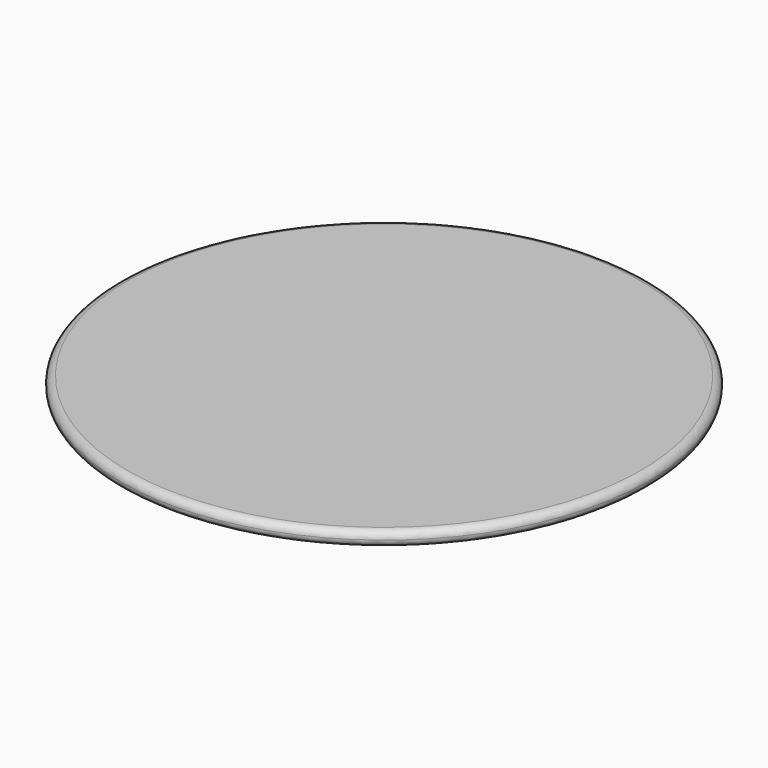
from build123d import *

# Parameters (mm, degrees)
F1_DEPTH = 31.75
F3_DEPTH = 19.05
F4_R     = 19.04999
F5_R     = 6.34999
F6_R     = 8.73125
F7_R     = 8.73125
F8_R     = 8.73125
F9_DEPTH = 19.05


# Not quite as in the source:
# - a fillet or chamfer is up to 0.001 mm smaller than in the source, because OpenCascade refuses the exact size


with BuildPart() as f1:
    # F0 (on Top) → F1 (new body)
    with BuildSketch(Plane.XY):
        with BuildLine():
            add(Edge.make_bspline(
                [(0, -228.6), (395.9468146102, -228.6), (197.9734073051, 114.3), (0, 457.2), (-197.9734073051, 114.3), (-395.9468146102, -228.6), (0, -228.6)],
                knots=[0, 0, 0, 2.0943951024, 2.0943951024, 4.1887902048, 4.1887902048, 6.2831853072, 6.2831853072, 6.2831853072], degree=2, weights=[1, 0.5, 1, 0.5, 1, 0.5, 1]))
        make_face()
    extrude(amount=F1_DEPTH)

    # F2 (on face) → F3 (cut)
    with BuildSketch(Plane(origin=(0, 0, 0), x_dir=(1, 0, 0), z_dir=(0, 0, -1))):
        with BuildLine():
            add(Edge.make_bspline(
                [(0, 228.6), (395.9468146102, 228.6), (197.9734073051, -114.3), (0, -457.2), (-197.9734073051, -114.3), (-395.9468146102, 228.6), (0, 228.6)],
                knots=[0, 0, 0, 2.0943951024, 2.0943951024, 4.1887902048, 4.1887902048, 6.2831853072, 6.2831853072, 6.2831853072], degree=2, weights=[1, 0.5, 1, 0.5, 1, 0.5, 1]))
        make_face()
        with BuildLine():
            ThreePointArc((-41.557586209, 123.9214253546), (-42.5423564602, 116.6976312088), (-45.4247989454, 110.0010276198))
            Line((-45.4247989454, 110.0010276198), (118.4713582711, 11.3214710191))
            ThreePointArc((118.4713582711, 11.3214710191), (148.8154396806, 23.4038030331), (168.5791455348, -2.5989267157))
            ThreePointArc((168.5791455348, -2.5989267157), (148.3370211672, -28.7298483188), (117.9760838338, -15.6614839614))
            Line((117.9760838338, -15.6614839614), (-49.4309976248, -108.2599413932))
            ThreePointArc((-49.4309976248, -108.2599413932), (-46.9156377226, -114.5771230065), (-46.0590593257, -121.3224986389))
            ThreePointArc((-46.0590593257, -121.3224986389), (-92.3039134421, -140.2296260962), (-72.5512848884, -94.3395436584))
            Line((-72.5512848884, -94.3395436584), (-69.0403606463, 96.9384703741))
            ThreePointArc((-69.0403606463, 96.9384703741), (-87.4522136664, 143.178779471), (-41.557586209, 123.9214253546))
        make_face(mode=Mode.SUBTRACT)
        with BuildLine():
            Line((118.4713582711, 11.3214710191), (-45.4247989454, 110.0010276198))
            ThreePointArc((-45.4247989454, 110.0010276198), (-55.4825289633, 100.3058636536), (-69.0403606463, 96.9384703741))
            Line((-69.0403606463, 96.9384703741), (-72.5512848884, -94.3395436584))
            ThreePointArc((-72.5512848884, -94.3395436584), (-59.1261615909, -98.2022113753), (-49.4309976248, -108.2599413932))
            Line((-49.4309976248, -108.2599413932), (117.9760838338, -15.6614839614))
            ThreePointArc((117.9760838338, -15.6614839614), (114.6086905542, -2.1036522784), (118.4713582711, 11.3214710191))
        make_face()
    extrude(amount=-F3_DEPTH, mode=Mode.SUBTRACT)

    # F4 (radius 19.05 in the source; OpenCascade refuses exactly that, so slightly less here)
    f4_edges = [f1.edges().sort_by_distance(p)[0] for p in [
        (-91.665373, -137.841823, 19.05),
        (165.207207, -10.463631, 19.05),
        (-73.541834, 148.305454, 19.05),
    ]]
    fillet(f4_edges, radius=F4_R)

    # F5 (radius 6.35 in the source; OpenCascade refuses exactly that, so slightly less here)
    f5_edges = [f1.edges().sort_by_distance(p)[0] for p in [
        (0, 228.6, 31.75),
        (0, 228.6, 19.05),
    ]]
    fillet(f5_edges, radius=F5_R)

    # F6 (on face) + F7 (on face) + F8 (on face) → F9 (cut)
    with BuildSketch(Plane(origin=(0, 0, 0), x_dir=(1, 0, 0), z_dir=(0, 0, -1))):
        with Locations((-68.545086209, 123.9214253546)):
            Circle(F6_R)
    with BuildSketch(Plane(origin=(0, 0, 0), x_dir=(1, 0, 0), z_dir=(0, 0, -1))):
        with Locations((141.5916455348, -2.5989267157)):
            Circle(F7_R)
    with BuildSketch(Plane(origin=(0, 0, 0), x_dir=(1, 0, 0), z_dir=(0, 0, -1))):
        with Locations((-73.0465593257, -121.3224986389)):
            Circle(F8_R)
    extrude(amount=-F9_DEPTH, mode=Mode.SUBTRACT)


solid = f1.part
